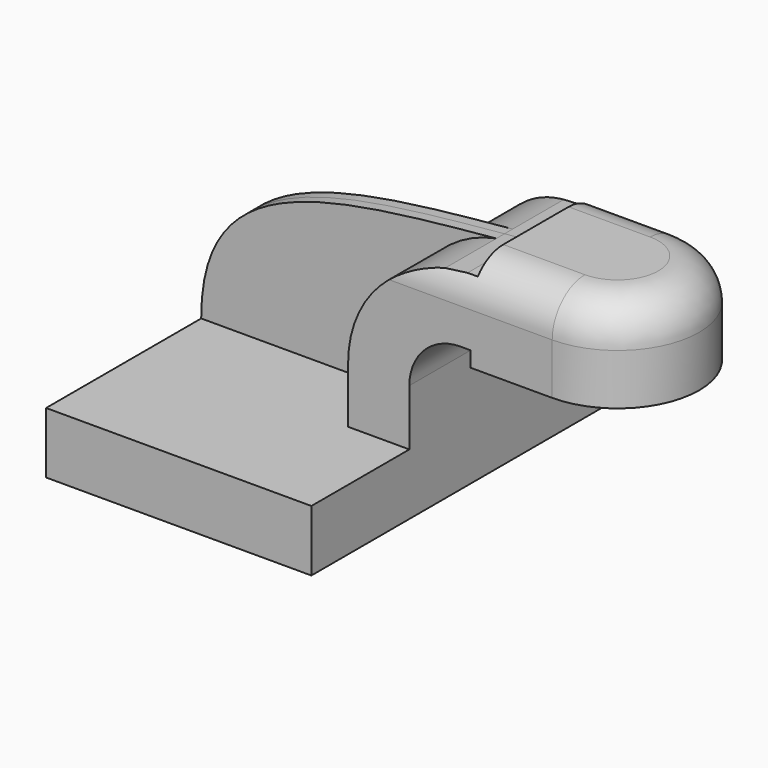
from build123d import *

# Parameters (mm, degrees)
F1_DEPTH = 63.5
F0_W     = 25.4
F0_H     = 19.05
F0_H_2   = 4.7498
F0_H_3   = 4.7752
F2_DEPTH = 25.4
F4_DEPTH = 3.175
F5_R     = 12.7


with BuildPart() as f1:
    # F0 (on Front) → F1 (new body, symmetric)
    with BuildSketch(Plane.XZ):
        Polygon((-41.275, -9.525), (41.275, -9.525), (41.275, 9.525), (22.225, 9.525), (-41.275, 9.525), align=None)
    extrude(amount=F1_DEPTH, both=True)

    # F0 (on Front) → F2 (join, symmetric)
    with BuildSketch(Plane.XZ):
        with BuildLine():
            Line((22.225, 9.525), (41.275, 9.525))
            Line((41.275, 9.525), (41.275, 27.0002))
            ThreePointArc((41.275, 27.0002), (45.9246798487, 38.2255201513), (57.15, 42.8752))
            Line((57.15, 42.8752), (60.325, 42.8752))
            Line((60.325, 42.8752), (60.325, 61.9252))
            Line((60.325, 61.9252), (57.15, 61.9252))
            add(Edge.make_bspline(
                [(50.5716827733, 61.3000741611), (52.7396972635, 61.5056461021), (54.9329690535, 61.7131439678), (57.15, 61.9252)],
                knots=[107.178919237, 107.178919237, 107.178919237, 107.178919237, 111.5045361635, 111.5045361635, 111.5045361635, 111.5045361635], degree=3))
            ThreePointArc((50.5716827733, 61.3000741611), (30.2287876003, 49.2488841842), (22.225, 27.0002))
            Line((22.225, 27.0002), (22.225, 9.525))
        make_face()
        with Locations((73.025, 52.4002)):
            Rectangle(F0_W, F0_H)
        with Locations((73.025, 64.3001)):
            Rectangle(F0_W, F0_H_2)
        with Locations((73.025, 40.4876)):
            Rectangle(F0_W, F0_H_3)
    extrude(amount=F2_DEPTH, both=True)

    # F0 (on Front) → F3 (revolve)
    with BuildSketch(Plane.XZ):
        Polygon((85.725, 61.9252), (85.725, 42.8752), (85.725, 38.1), (111.125, 38.1), (111.125, 66.675), (85.725, 66.675), align=None)
    revolve(axis=Axis((85.725, 0, 52.3875), (0, 0, 1)))

    # F0 (on Front) → F4 (join, symmetric)
    with BuildSketch(Plane.XZ):
        with BuildLine():
            add(Edge.make_bspline(
                [(-41.275, 9.525), (-41.358874461, 52.2952599857), (-3.1467703164, 56.2064704424), (50.5716827733, 61.3000741611)],
                knots=[0, 0, 0, 0, 107.178919237, 107.178919237, 107.178919237, 107.178919237], degree=3))
            Line((-41.275, 9.525), (22.225, 9.525))
            Line((22.225, 9.525), (22.225, 27.0002))
            ThreePointArc((22.225, 27.0002), (30.2287876003, 49.2488841842), (50.5716827733, 61.3000741611))
        make_face()
    extrude(amount=F4_DEPTH, both=True)

    # F5
    f5_edges = [f1.edges().sort_by_distance(p)[0] for p in [
        (85.725, 25.4, 52.3875),
        (73.025, 25.4, 66.675),
        (73.025, -25.4, 66.675),
        (111.125, 0, 66.675),
    ]]
    fillet(f5_edges, radius=F5_R)


solid = f1.part
